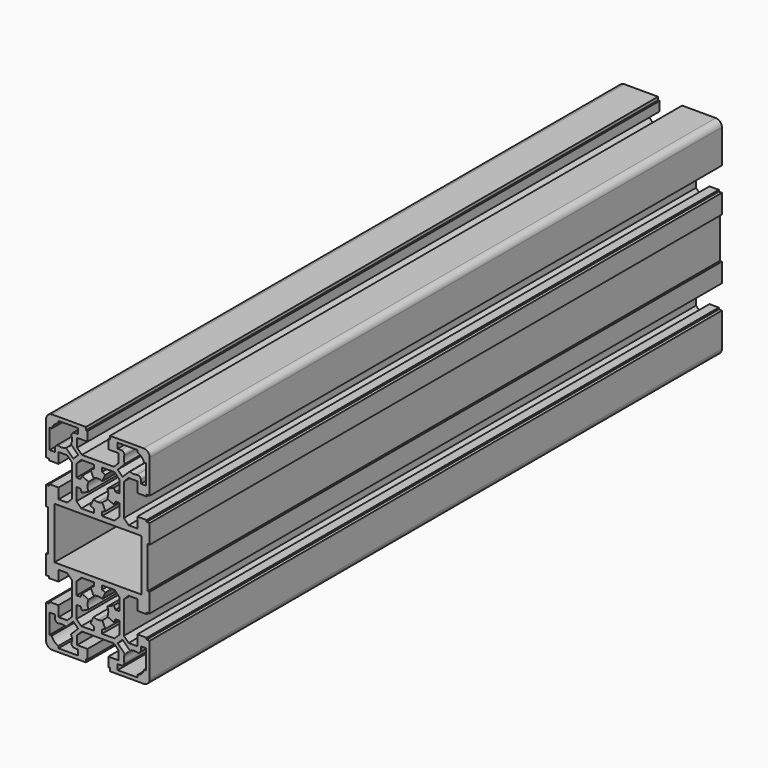
from build123d import *

# Parameters (mm, degrees)
F3_DEPTH = 345


# Not quite as in the source:
# - ends of sketch curves that miss each other by under 0.0002 mm in the source are joined


with BuildPart() as f3:
    # F2 (on Front) → F3 (new body)
    with BuildSketch(Plane.XZ):
        with BuildLine():
            Line((21.000169, 12.449667), (21.000169, -0.000333))
            Line((21.000169, -0.000333), (24.000169, -0.000333))
            Line((24.000169, -0.000333), (24.000169, 9.999667))
            Line((24.000169, 9.999667), (25.000169, 9.999667))
            Line((25.000169, 9.999667), (25.000169, 19.199667))
            Line((25.000169, 19.199667), (23.500169, 19.199667))
            Line((23.500169, 19.199667), (23.500169, 19.999667))
            Line((23.500169, 19.999667), (19.000169, 19.999667))
            Line((19.000169, 19.999667), (19.000169, 14.949667))
            Line((19.000169, 14.949667), (14.800169, 14.949667))
            Line((14.800169, 14.949667), (12.500169, 17.249667))
            Line((12.500169, 17.249667), (12.500169, 32.749667))
            Line((12.500169, 32.749667), (14.800169, 35.049667))
            Line((14.800169, 35.049667), (19.000169, 35.049667))
            Line((19.000169, 35.049667), (19.000169, 29.999667))
            Line((19.000169, 29.999667), (23.500169, 29.999667))
            Line((23.500169, 29.999667), (23.500169, 30.799667))
            Line((23.500169, 30.799667), (25.000169, 30.799667))
            Line((25.000169, 30.799667), (25.000169, 46.999667))
            ThreePointArc((25.000169, 46.999667), (24.1214893436, 49.1209873436), (22.000169, 49.999667))
            Line((22.000169, 49.999667), (5.800169, 49.999667))
            Line((5.800169, 49.999667), (5.800169, 48.499667))
            Line((5.800169, 48.499667), (5.000169, 48.499667))
            Line((5.000169, 48.499667), (5.000169, 43.999667))
            Line((5.000169, 43.999667), (10.050169, 43.999667))
            Line((10.050169, 43.999667), (10.050169, 39.799667))
            Line((10.050169, 39.799667), (7.750169, 37.499667))
            Line((7.750169, 37.499667), (0.000169, 37.499667))
            Line((0.000169, 37.499667), (0.000169, 29.999667))
            ThreePointArc((0.000169, 29.999667), (1.0823669197, 29.8811470688), (2.1132600303, 29.531206065))
            Line((2.11326, 29.531206), (3.592424, 32.703283))
            Line((3.592424, 32.703283), (2.000169, 33.445764))
            Line((2.000169, 33.445764), (2.000169, 35.299667))
            Line((2.000169, 35.299667), (8.012449, 35.299667))
            Line((8.012449, 35.299667), (10.300169, 33.011947))
            Line((10.300169, 33.011947), (10.300169, 26.999667))
            Line((10.300169, 26.999667), (8.446266, 26.999667))
            Line((8.446266, 26.999667), (7.703785, 28.591922))
            Line((7.703785, 28.591922), (4.531708, 27.112758))
            ThreePointArc((4.531708065, 27.1127580303), (5.000169, 24.999667), (4.531708065, 22.8865759697))
            Line((4.531708, 22.886576), (7.703785, 21.407412))
            Line((7.703785, 21.407412), (8.446266, 22.999667))
            Line((8.446266, 22.999667), (10.300169, 22.999667))
            Line((10.300169, 22.999667), (10.300169, 16.987387))
            Line((10.300169, 16.987387), (8.012449, 14.699667))
            Line((8.012449, 14.699667), (2.000169, 14.699667))
            Line((2.000169, 14.699667), (2.000169, 16.55357))
            Line((2.000169, 16.55357), (3.592424, 17.296051))
            Line((3.592424, 17.296051), (2.11326, 20.468128))
            ThreePointArc((2.1132600303, 20.468127935), (1.0823669197, 20.1181869312), (0.000169, 19.999667))
            Line((0.000169, 19.999667), (0.000169, 12.449667))
            Line((0.000169, 12.449667), (21.000169, 12.449667))
        make_face()
        with BuildLine():
            Line((20.700169, 34.499667), (20.700169, 36.225912))
            ThreePointArc((20.700169, 36.225912), (20.1116343558, 37.41722678), (18.8078611265, 37.6737015332))
            ThreePointArc((18.8078611265, 37.6737015332), (17.1448966414, 37.5123048163), (15.5216018999, 37.9077967677))
            ThreePointArc((15.5216018999, 37.9077967677), (15.3464434299, 37.9269271737), (15.1907559656, 37.8444170344))
            Line((15.1907559656, 37.8444170344), (11.884862, 34.538523))
            Line((11.884862, 34.538523), (9.539025, 36.88436))
            Line((9.539025, 36.88436), (12.844919, 40.190254))
            ThreePointArc((12.844919, 40.190254), (12.9274291737, 40.3459414299), (12.9082991899, 40.5211000818))
            ThreePointArc((12.9082991899, 40.5211000818), (12.5128068163, 42.1443946414), (12.6742036668, 43.8073590903))
            ThreePointArc((12.6742036668, 43.8073590903), (12.41772878, 45.1111323558), (11.226414, 45.699667))
            Line((11.226414, 45.699667), (9.500169, 45.699667))
            Line((9.500169, 45.699667), (9.500169, 48.299667))
            Line((9.500169, 48.299667), (19.000169, 48.299667))
            Line((19.000169, 48.299667), (19.000169, 47.269363))
            ThreePointArc((19.000169, 47.269363), (21.0357029059, 46.0352009059), (22.2698650064, 43.999667002))
            Line((22.2698650064, 43.999667002), (23.300169, 43.999667))
            Line((23.300169, 43.999667), (23.300169, 34.499667))
            Line((23.300169, 34.499667), (20.700169, 34.499667))
        make_face(mode=Mode.SUBTRACT)
        with BuildLine():
            Line((-23.999831, -0.000333), (-20.999831, -0.000333))
            Line((-20.999831, -0.000333), (-20.999831, 12.449667))
            Line((-20.999831, 12.449667), (0.000169, 12.449667))
            Line((0.000169, 12.449667), (0.000169, 19.999667))
            ThreePointArc((0.000169, 19.999667), (-1.0820289197, 20.1181869312), (-2.1129220303, 20.468127935))
            Line((-2.112922, 20.468128), (-3.592086, 17.296051))
            Line((-3.592086, 17.296051), (-1.999831, 16.55357))
            Line((-1.999831, 16.55357), (-1.999831, 14.699667))
            Line((-1.999831, 14.699667), (-8.012111, 14.699667))
            Line((-8.012111, 14.699667), (-10.299831, 16.987387))
            Line((-10.299831, 16.987387), (-10.299831, 22.999667))
            Line((-10.299831, 22.999667), (-8.445928, 22.999667))
            Line((-8.445928, 22.999667), (-7.703447, 21.407412))
            Line((-7.703447, 21.407412), (-4.53137, 22.886576))
            ThreePointArc((-4.531370065, 22.8865759697), (-4.999831, 24.999667), (-4.531370065, 27.1127580303))
            Line((-4.53137, 27.112758), (-7.703447, 28.591922))
            Line((-7.703447, 28.591922), (-8.445928, 26.999667))
            Line((-8.445928, 26.999667), (-10.299831, 26.999667))
            Line((-10.299831, 26.999667), (-10.299831, 33.011947))
            Line((-10.299831, 33.011947), (-8.012111, 35.299667))
            Line((-8.012111, 35.299667), (-1.999831, 35.299667))
            Line((-1.999831, 35.299667), (-1.999831, 33.445764))
            Line((-1.999831, 33.445764), (-3.592086, 32.703283))
            Line((-3.592086, 32.703283), (-2.112922, 29.531206))
            ThreePointArc((-2.1129220303, 29.531206065), (-1.0820289197, 29.8811470688), (0.000169, 29.999667))
            Line((0.000169, 29.999667), (0.000169, 37.499667))
            Line((0.000169, 37.499667), (-7.749831, 37.499667))
            Line((-7.749831, 37.499667), (-10.049831, 39.799667))
            Line((-10.049831, 39.799667), (-10.049831, 43.999667))
            Line((-10.049831, 43.999667), (-4.999831, 43.999667))
            Line((-4.999831, 43.999667), (-4.999831, 48.499667))
            Line((-4.999831, 48.499667), (-5.799831, 48.499667))
            Line((-5.799831, 48.499667), (-5.799831, 49.999667))
            Line((-5.799831, 49.999667), (-21.999831, 49.999667))
            ThreePointArc((-21.999831, 49.999667), (-24.1211513436, 49.1209873436), (-24.999831, 46.999667))
            Line((-24.999831, 46.999667), (-24.999831, 30.799667))
            Line((-24.999831, 30.799667), (-23.499831, 30.799667))
            Line((-23.499831, 30.799667), (-23.499831, 29.999667))
            Line((-23.499831, 29.999667), (-18.999831, 29.999667))
            Line((-18.999831, 29.999667), (-18.999831, 35.049667))
            Line((-18.999831, 35.049667), (-14.799831, 35.049667))
            Line((-14.799831, 35.049667), (-12.499831, 32.749667))
            Line((-12.499831, 32.749667), (-12.499831, 17.249667))
            Line((-12.499831, 17.249667), (-14.799831, 14.949667))
            Line((-14.799831, 14.949667), (-18.999831, 14.949667))
            Line((-18.999831, 14.949667), (-18.999831, 19.999667))
            Line((-18.999831, 19.999667), (-23.499831, 19.999667))
            Line((-23.499831, 19.999667), (-23.499831, 19.199667))
            Line((-23.499831, 19.199667), (-24.999831, 19.199667))
            Line((-24.999831, 19.199667), (-24.999831, 9.999667))
            Line((-24.999831, 9.999667), (-23.999831, 9.999667))
            Line((-23.999831, 9.999667), (-23.999831, -0.000333))
        make_face()
        with BuildLine():
            ThreePointArc((-15.5212638999, 37.9077967677), (-17.1445586414, 37.5123048163), (-18.8075230903, 37.6737016668))
            ThreePointArc((-18.8075230903, 37.6737016668), (-20.1112963558, 37.41722678), (-20.699831, 36.225912))
            Line((-20.699831, 36.225912), (-20.699831, 34.499667))
            Line((-20.699831, 34.499667), (-23.299831, 34.499667))
            Line((-23.299831, 34.499667), (-23.299831, 43.999667))
            Line((-23.299831, 43.999667), (-22.269527, 43.999667))
            ThreePointArc((-22.269527, 43.999667), (-21.0353649059, 46.0352009059), (-18.999831002, 47.2693630064))
            Line((-18.999831002, 47.2693630064), (-18.999831, 48.299667))
            Line((-18.999831, 48.299667), (-9.499831, 48.299667))
            Line((-9.499831, 48.299667), (-9.499831, 45.699667))
            Line((-9.499831, 45.699667), (-11.226076, 45.699667))
            ThreePointArc((-11.226076, 45.699667), (-12.41739078, 45.1111323558), (-12.6738655332, 43.8073591265))
            ThreePointArc((-12.6738655332, 43.8073591265), (-12.5124688163, 42.1443946414), (-12.9079607677, 40.5210998999))
            ThreePointArc((-12.9079607677, 40.5210998999), (-12.9270911737, 40.3459414299), (-12.8445810344, 40.1902539656))
            Line((-12.8445810344, 40.1902539656), (-9.538687, 36.88436))
            Line((-9.538687, 36.88436), (-11.884524, 34.538523))
            Line((-11.884524, 34.538523), (-15.190418, 37.844417))
            ThreePointArc((-15.190418, 37.844417), (-15.3461054299, 37.9269271737), (-15.5212638999, 37.9077967677))
        make_face(mode=Mode.SUBTRACT)
        with BuildLine():
            Line((5.800169, -50.000333), (22.000169, -50.000333))
            ThreePointArc((22.000169, -50.000333), (24.1214893436, -49.1216533436), (25.000169, -47.000333))
            Line((25.000169, -47.000333), (25.000169, -30.800333))
            Line((25.000169, -30.800333), (23.500169, -30.800333))
            Line((23.500169, -30.800333), (23.500169, -30.000333))
            Line((23.500169, -30.000333), (19.000169, -30.000333))
            Line((19.000169, -30.000333), (19.000169, -35.050333))
            Line((19.000169, -35.050333), (14.800169, -35.050333))
            Line((14.800169, -35.050333), (12.500169, -32.750333))
            Line((12.500169, -32.750333), (12.500169, -17.250333))
            Line((12.500169, -17.250333), (14.800169, -14.950333))
            Line((14.800169, -14.950333), (19.000169, -14.950333))
            Line((19.000169, -14.950333), (19.000169, -20.000333))
            Line((19.000169, -20.000333), (23.500169, -20.000333))
            Line((23.500169, -20.000333), (23.500169, -19.200333))
            Line((23.500169, -19.200333), (25.000169, -19.200333))
            Line((25.000169, -19.200333), (25.000169, -10.000333))
            Line((25.000169, -10.000333), (24.000169, -10.000333))
            Line((24.000169, -10.000333), (24.000169, -0.000333))
            Line((24.000169, -0.000333), (21.000169, -0.000333))
            Line((21.000169, -0.000333), (21.000169, -12.450333))
            Line((21.000169, -12.450333), (0.000169, -12.450333))
            Line((0.000169, -12.450333), (0.000169, -20.000333))
            ThreePointArc((0.000169, -20.000333), (1.0823669197, -20.1188529312), (2.1132600303, -20.468793935))
            Line((2.11326, -20.468794), (3.592424, -17.296717))
            Line((3.592424, -17.296717), (2.000169, -16.554236))
            Line((2.000169, -16.554236), (2.000169, -14.700333))
            Line((2.000169, -14.700333), (8.012449, -14.700333))
            Line((8.012449, -14.700333), (10.300169, -16.988053))
            Line((10.300169, -16.988053), (10.300169, -23.000333))
            Line((10.300169, -23.000333), (8.446266, -23.000333))
            Line((8.446266, -23.000333), (7.703785, -21.408078))
            Line((7.703785, -21.408078), (4.531708, -22.887242))
            ThreePointArc((4.531708065, -22.8872419697), (5.000169, -25.000333), (4.531708065, -27.1134240303))
            Line((4.531708, -27.113424), (7.703785, -28.592588))
            Line((7.703785, -28.592588), (8.446266, -27.000333))
            Line((8.446266, -27.000333), (10.300169, -27.000333))
            Line((10.300169, -27.000333), (10.300169, -33.012613))
            Line((10.300169, -33.012613), (8.012449, -35.300333))
            Line((8.012449, -35.300333), (2.000169, -35.300333))
            Line((2.000169, -35.300333), (2.000169, -33.44643))
            Line((2.000169, -33.44643), (3.592424, -32.703949))
            Line((3.592424, -32.703949), (2.11326, -29.531872))
            ThreePointArc((2.1132600303, -29.531872065), (1.0823669197, -29.8818130688), (0.000169, -30.000333))
            Line((0.000169, -30.000333), (0.000169, -37.500333))
            Line((0.000169, -37.500333), (7.750169, -37.500333))
            Line((7.750169, -37.500333), (10.050169, -39.800333))
            Line((10.050169, -39.800333), (10.050169, -44.000333))
            Line((10.050169, -44.000333), (5.000169, -44.000333))
            Line((5.000169, -44.000333), (5.000169, -48.500333))
            Line((5.000169, -48.500333), (5.800169, -48.500333))
            Line((5.800169, -48.500333), (5.800169, -50.000333))
        make_face()
        with BuildLine():
            ThreePointArc((12.6742036668, -43.8080250903), (12.5128068163, -42.1450606414), (12.9082987677, -40.5217658999))
            ThreePointArc((12.9082987677, -40.5217658999), (12.9274291737, -40.3466074299), (12.8449190344, -40.1909199656))
            Line((12.8449190344, -40.1909199656), (9.539025, -36.885026))
            Line((9.539025, -36.885026), (11.884862, -34.539189))
            Line((11.884862, -34.539189), (15.190756, -37.845083))
            ThreePointArc((15.190756, -37.845083), (15.3464434299, -37.9275931737), (15.5216020818, -37.9084631899))
            ThreePointArc((15.5216020818, -37.9084631899), (17.1448966414, -37.5129708163), (18.8078610903, -37.6743676668))
            ThreePointArc((18.8078610903, -37.6743676668), (20.1116343558, -37.41789278), (20.700169, -36.226578))
            Line((20.700169, -36.226578), (20.700169, -34.500333))
            Line((20.700169, -34.500333), (23.300169, -34.500333))
            Line((23.300169, -34.500333), (23.300169, -44.000333))
            Line((23.300169, -44.000333), (22.269865, -44.000333))
            ThreePointArc((22.269865, -44.000333), (21.0357029059, -46.0358669059), (19.000169002, -47.2700290064))
            Line((19.000169002, -47.2700290064), (19.000169, -48.300333))
            Line((19.000169, -48.300333), (9.500169, -48.300333))
            Line((9.500169, -48.300333), (9.500169, -45.700333))
            Line((9.500169, -45.700333), (11.226414, -45.700333))
            ThreePointArc((11.226414, -45.700333), (12.41772878, -45.1117983558), (12.6742036668, -43.8080250903))
        make_face(mode=Mode.SUBTRACT)
        with BuildLine():
            Line((-7.749831, -37.500333), (0.000169, -37.500333))
            Line((0.000169, -37.500333), (0.000169, -30.000333))
            ThreePointArc((0.000169, -30.000333), (-1.0820289197, -29.8818130688), (-2.1129220303, -29.531872065))
            Line((-2.112922, -29.531872), (-3.592086, -32.703949))
            Line((-3.592086, -32.703949), (-1.999831, -33.44643))
            Line((-1.999831, -33.44643), (-1.999831, -35.300333))
            Line((-1.999831, -35.300333), (-8.012111, -35.300333))
            Line((-8.012111, -35.300333), (-10.299831, -33.012613))
            Line((-10.299831, -33.012613), (-10.299831, -27.000333))
            Line((-10.299831, -27.000333), (-8.445928, -27.000333))
            Line((-8.445928, -27.000333), (-7.703447, -28.592588))
            Line((-7.703447, -28.592588), (-4.53137, -27.113424))
            ThreePointArc((-4.531370065, -27.1134240303), (-4.999831, -25.000333), (-4.531370065, -22.8872419697))
            Line((-4.53137, -22.887242), (-7.703447, -21.408078))
            Line((-7.703447, -21.408078), (-8.445928, -23.000333))
            Line((-8.445928, -23.000333), (-10.299831, -23.000333))
            Line((-10.299831, -23.000333), (-10.299831, -16.988053))
            Line((-10.299831, -16.988053), (-8.012111, -14.700333))
            Line((-8.012111, -14.700333), (-1.999831, -14.700333))
            Line((-1.999831, -14.700333), (-1.999831, -16.554236))
            Line((-1.999831, -16.554236), (-3.592086, -17.296717))
            Line((-3.592086, -17.296717), (-2.112922, -20.468794))
            ThreePointArc((-2.1129220303, -20.468793935), (-1.0820289197, -20.1188529312), (0.000169, -20.000333))
            Line((0.000169, -20.000333), (0.000169, -12.450333))
            Line((0.000169, -12.450333), (-20.999831, -12.450333))
            Line((-20.999831, -12.450333), (-20.999831, -0.000333))
            Line((-20.999831, -0.000333), (-23.999831, -0.000333))
            Line((-23.999831, -0.000333), (-23.999831, -10.000333))
            Line((-23.999831, -10.000333), (-24.999831, -10.000333))
            Line((-24.999831, -10.000333), (-24.999831, -19.200333))
            Line((-24.999831, -19.200333), (-23.499831, -19.200333))
            Line((-23.499831, -19.200333), (-23.499831, -20.000333))
            Line((-23.499831, -20.000333), (-18.999831, -20.000333))
            Line((-18.999831, -20.000333), (-18.999831, -14.950333))
            Line((-18.999831, -14.950333), (-14.799831, -14.950333))
            Line((-14.799831, -14.950333), (-12.499831, -17.250333))
            Line((-12.499831, -17.250333), (-12.499831, -32.750333))
            Line((-12.499831, -32.750333), (-14.799831, -35.050333))
            Line((-14.799831, -35.050333), (-18.999831, -35.050333))
            Line((-18.999831, -35.050333), (-18.999831, -30.000333))
            Line((-18.999831, -30.000333), (-23.499831, -30.000333))
            Line((-23.499831, -30.000333), (-23.499831, -30.800333))
            Line((-23.499831, -30.800333), (-24.999831, -30.800333))
            Line((-24.999831, -30.800333), (-24.999831, -47.000333))
            ThreePointArc((-24.999831, -47.000333), (-24.1211513436, -49.1216533436), (-21.999831, -50.000333))
            Line((-21.999831, -50.000333), (-5.799831, -50.000333))
            Line((-5.799831, -50.000333), (-5.799831, -48.500333))
            Line((-5.799831, -48.500333), (-4.999831, -48.500333))
            Line((-4.999831, -48.500333), (-4.999831, -44.000333))
            Line((-4.999831, -44.000333), (-10.049831, -44.000333))
            Line((-10.049831, -44.000333), (-10.049831, -39.800333))
            Line((-10.049831, -39.800333), (-7.749831, -37.500333))
        make_face()
        with BuildLine():
            ThreePointArc((-12.9079607677, -40.5217658999), (-12.5124688163, -42.1450606414), (-12.6738656668, -43.8080250903))
            ThreePointArc((-12.6738656668, -43.8080250903), (-12.41739078, -45.1117983558), (-11.226076, -45.700333))
            Line((-11.226076, -45.700333), (-9.499831, -45.700333))
            Line((-9.499831, -45.700333), (-9.499831, -48.300333))
            Line((-9.499831, -48.300333), (-18.999831, -48.300333))
            Line((-18.999831, -48.300333), (-18.999831, -47.270029))
            ThreePointArc((-18.999831, -47.270029), (-21.0353649059, -46.0358669059), (-22.2695270064, -44.000333002))
            Line((-22.2695270064, -44.000333002), (-23.299831, -44.000333))
            Line((-23.299831, -44.000333), (-23.299831, -34.500333))
            Line((-23.299831, -34.500333), (-20.699831, -34.500333))
            Line((-20.699831, -34.500333), (-20.699831, -36.226578))
            ThreePointArc((-20.699831, -36.226578), (-20.1112963558, -37.41789278), (-18.8075231265, -37.6743675332))
            ThreePointArc((-18.8075231265, -37.6743675332), (-17.1445586414, -37.5129708163), (-15.5212638999, -37.9084627677))
            ThreePointArc((-15.5212638999, -37.9084627677), (-15.3461054299, -37.9275931737), (-15.1904179656, -37.8450830344))
            Line((-15.1904179656, -37.8450830344), (-11.884524, -34.539189))
            Line((-11.884524, -34.539189), (-9.538687, -36.885026))
            Line((-9.538687, -36.885026), (-12.844581, -40.19092))
            ThreePointArc((-12.844581, -40.19092), (-12.9270911737, -40.3466074299), (-12.9079607677, -40.5217658999))
        make_face(mode=Mode.SUBTRACT)
    extrude(amount=-F3_DEPTH)


solid = f3.part
